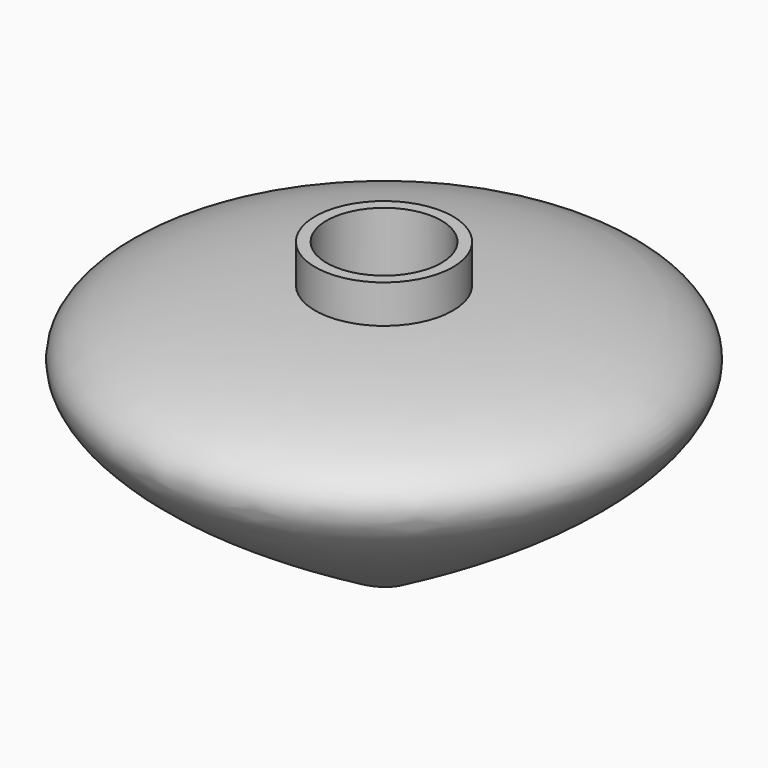
from build123d import *

# Parameters (mm, degrees)
F2_R     = 4.7625
F3_DEPTH = 9.525
F4_R     = 2.2225
F5_DEPTH = 14.605


# Not quite as in the source:
# - a feature names something its author has since deleted; it is built from what else it names


with BuildPart() as f1:
    # F0 (on Front) → F1 (revolve)
    with BuildSketch(Plane.XZ):
        with BuildLine():
            Line((0, 25.4), (0, 0))
            add(Edge.make_bspline(
                [(0, 0), (11.4623733169, 6.6295765693), (30.9367325307, 18.1147399727), (14.1349324056, 21.8956786186), (5.715, 22.225)],
                knots=[0, 0, 0, 0, 0.5612625766, 1, 1, 1, 1], degree=3))
            Line((5.715, 22.225), (5.715, 25.4))
            Line((5.715, 25.4), (0, 25.4))
        make_face()
    revolve(axis=Axis((0, 0, 12.7), (0, 0, -1)))

    # F2 (on face) → F3 (cut)
    with BuildSketch(Plane.XY.offset(25.4)):
        Circle(F2_R)
    extrude(amount=-F3_DEPTH, mode=Mode.SUBTRACT)

    # F4 (on Top) → F5 (cut)
    with BuildSketch(Plane.XY):
        with Locations((0, -0.9156785202)):
            Circle(F4_R)
    extrude(amount=F5_DEPTH, mode=Mode.SUBTRACT)


solid = f1.part
